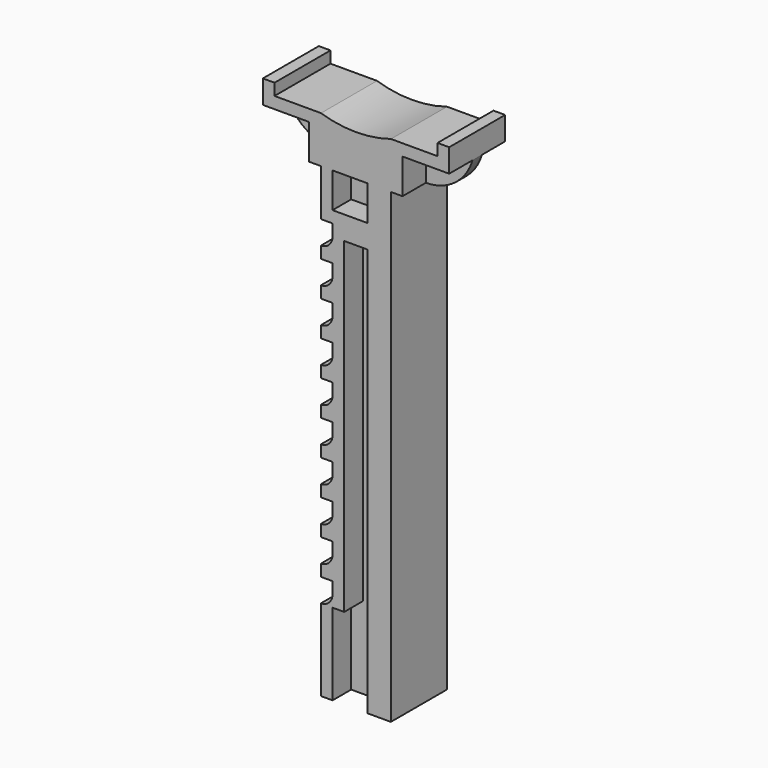
from build123d import *

# Parameters (mm, degrees)
F1_DEPTH  = 30
F2_R      = 4.99999
F3_W      = 15
F3_H      = 15
F4_DEPTH  = 10
F5_W      = 15
F5_H      = 15
F6_DEPTH  = 10
F8_DEPTH  = 30
F10_DEPTH = 17.5
F12_DEPTH = 12.5
F14_DEPTH = 30


# Not quite as in the source:
# - a fillet or chamfer is up to 0.001 mm smaller than in the source, because OpenCascade refuses the exact size


with BuildPart() as f1:
    # F0 (on Front) → F1 (new body)
    with BuildSketch(Plane.XZ):
        Polygon((-25, -42.9761418055), (-25, -77.9761418055), (5, -77.9761418055), (5, 122.0238581945), (10, 122.0238581945), (10, 137.0238581945), (-30, 137.0238581945), (-30, 122.0238581945), (-25, 122.0238581945), (-25, 102.0238581945), (-20, 102.0238581945), (-20, 92.0238581945), (-25, 92.0238581945), (-25, 87.0238581945), (-20, 87.0238581945), (-20, 77.0238581945), (-25, 77.0238581945), (-25, 72.0238581945), (-20, 72.0238581945), (-20, 62.0238581945), (-25, 62.0238581945), (-25, 57.0238581945), (-20, 57.0238581945), (-20, 47.0238581945), (-25, 47.0238581945), (-25, 42.0238581945), (-20, 42.0238581945), (-20, 32.0238581945), (-25, 32.0238581945), (-25, 27.0238581945), (-20, 27.0238581945), (-20, 17.0238581945), (-25, 17.0238581945), (-25, 12.0238581945), (-20, 12.0238581945), (-20, 2.0238581945), (-25, 2.0238581945), (-25, -2.9761418055), (-20, -2.9761418055), (-20, -12.9761418055), (-25, -12.9761418055), (-25, -17.9761418055), (-20, -17.9761418055), (-20, -27.9761418055), (-25, -27.9761418055), (-25, -32.9761418055), (-20, -32.9761418055), (-20, -42.9761418055), align=None)
    extrude(amount=F1_DEPTH)

    # F2 (radius 5 in the source; OpenCascade refuses exactly that, so slightly less here)
    f2_edges = [f1.edges().sort_by_distance(p)[0] for p in [
        (-20, -15, 92.023858),
        (-20, -15, 77.023858),
        (-20, -15, 62.023858),
        (-20, -15, 47.023858),
        (-20, -15, 32.023858),
        (-20, -15, 17.023858),
        (-20, -15, 2.023858),
        (-20, -15, -12.976142),
        (-20, -15, -27.976142),
        (-20, -15, -42.976142),
    ]]
    fillet(f2_edges, radius=F2_R)

    # F3 (on face) → F4 (cut)
    with BuildSketch(Plane.XZ.offset(30)):
        Polygon((-15, -42.9761418055), (-20, -42.9761418055), (-20, -77.9761418055), (-5, -77.9761418055), (-5, 97.0238581945), (-15, 97.0238581945), align=None)
        with Locations((-12.5, 114.5238581945)):
            Rectangle(F3_W, F3_H)
    extrude(amount=-F4_DEPTH, mode=Mode.SUBTRACT)

    # F5 (on face) → F6 (cut)
    with BuildSketch(Plane(origin=(0, 0, 0), x_dir=(-1, 0, 0), z_dir=(0, 1, 0))):
        Polygon((20, -77.9761418055), (20, -42.9761418055), (15, -42.9761418055), (15, 96.101924777), (5, 96.101924777), (5, -77.9761418055), align=None)
        with Locations((12.5, 114.5238581945)):
            Rectangle(F5_W, F5_H)
    extrude(amount=-F6_DEPTH, mode=Mode.SUBTRACT)

    # F7 (on face) → F8 (join)
    with BuildSketch(Plane(origin=(0, 0, 0), x_dir=(-1, 0, 0), z_dir=(0, 1, 0))):
        Polygon((-30, 147.0238581945), (-30, 137.0238581945), (49.8739863932, 137.0238581945), (49.8739863932, 147.0238581945), (44.8739863932, 147.0238581945), (44.8739863932, 142.0238581945), (-25, 142.0238581945), (-25, 147.0238581945), align=None)
    extrude(amount=-F8_DEPTH)

    # F9 (on face) → F10 (join)
    with BuildSketch(Plane.XZ.offset(30)):
        with BuildLine():
            Line((-30, 137.0238581945), (-49.8739863932, 137.0238581945))
            ThreePointArc((-49.8739863932, 137.0238581945), (-42.4496519545, 126.1947551301), (-30, 122.0238581945))
            Line((-30, 122.0238581945), (-30, 137.0238581945))
        make_face()
        with BuildLine():
            ThreePointArc((10, 122.0238581945), (22.5, 126.1905248612), (30, 137.0238581945))
            Line((30, 137.0238581945), (10, 137.0238581945))
            Line((10, 137.0238581945), (10, 122.0238581945))
        make_face()
    extrude(amount=-F10_DEPTH)

    # F11 (on face) → F12 (cut)
    with BuildSketch(Plane.XZ.offset(30)):
        with BuildLine():
            Line((-30, 137.0238581945), (-49.8739863932, 137.0238581945))
            ThreePointArc((-49.8739863932, 137.0238581945), (-42.4496519545, 126.1947551301), (-30, 122.0238581945))
            Line((-30, 122.0238581945), (-30, 137.0238581945))
        make_face()
        with BuildLine():
            Line((10, 137.0238581945), (10, 122.0238581945))
            ThreePointArc((10, 122.0238581945), (22.5, 126.1905248612), (30, 137.0238581945))
            Line((30, 137.0238581945), (10, 137.0238581945))
        make_face()
    extrude(amount=-F12_DEPTH, mode=Mode.SUBTRACT)

    # F13 (on face) → F14 (cut)
    with BuildSketch(Plane(origin=(0, 0, 0), x_dir=(-1, 0, 0), z_dir=(0, 1, 0))):
        with BuildLine():
            Line((24.9369931966, 142.0238581945), (9.9369931966, 142.0238581945))
            Line((9.9369931966, 142.0238581945), (-5.0630068034, 142.0238581945))
            ThreePointArc((-5.0630068034, 142.0238581945), (9.9369931966, 139.7208182654), (24.9369931966, 142.0238581945))
        make_face()
    extrude(amount=-F14_DEPTH, mode=Mode.SUBTRACT)


solid = f1.part
